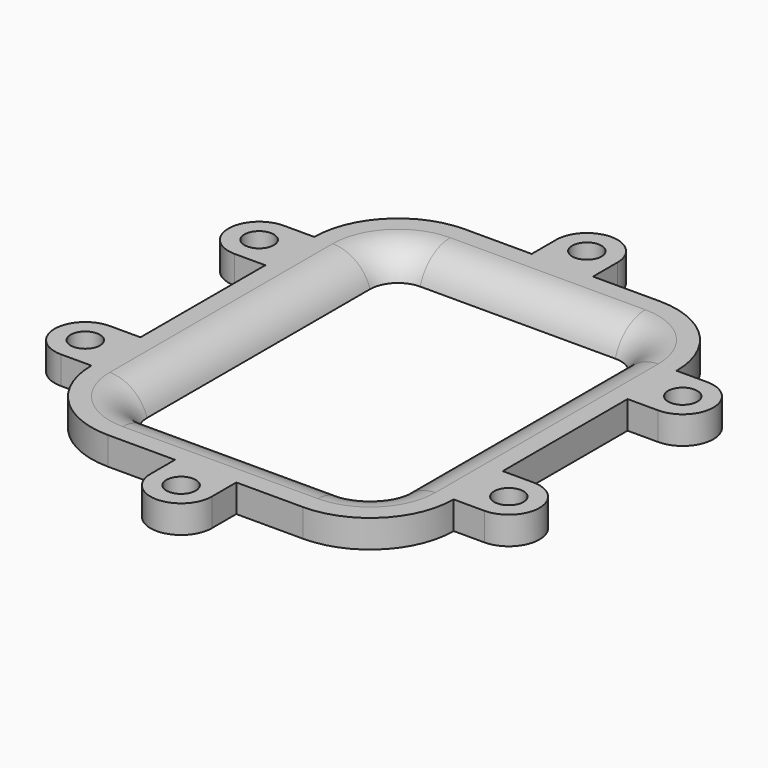
from build123d import *

# Parameters (mm, degrees)
F1_DEPTH     = 5
F3_D         = 5.25
F3_DEPTH     = 40
F3_TIP       = 1.5772591249
F4_T1_DEPTH  = 50
F4_T3_DEPTH  = 35
F4_T6_ANGLE  = 90
F4_T8_ANGLE  = 90
F4_T10_ANGLE = 90
F4_T12_ANGLE = 90


# Not quite as in the source:
# - a fillet or chamfer that OpenCascade refuses, or shapes differently, is made with other operations: its cross-section is extruded or revolved along the edge and cut away or added


with BuildPart() as f1:
    # F0 (on Top) → F1 (new body)
    with BuildSketch(Plane.XY):
        with BuildLine():
            Line((-38, -25), (-32.5, -25))
            ThreePointArc((-32.5, -25), (-28.1066017178, -35.6066017178), (-17.5, -40))
            Line((-17.5, -40), (-5.5, -40))
            Line((-5.5, -40), (-5.5, -45.5))
            ThreePointArc((-5.5, -45.5), (0, -51), (5.5, -45.5))
            Line((5.5, -45.5), (5.5, -40))
            Line((5.5, -40), (17.5, -40))
            ThreePointArc((17.5, -40), (28.1066017178, -35.6066017178), (32.5, -25))
            Line((32.5, -25), (38, -25))
            ThreePointArc((38, -25), (43.5, -19.5), (38, -14))
            Line((38, -14), (32.5, -14))
            Line((32.5, -14), (32.5, 14))
            Line((32.5, 14), (38, 14))
            ThreePointArc((38, 14), (43.5, 19.5), (38, 25))
            Line((38, 25), (32.5, 25))
            ThreePointArc((32.5, 25), (28.1066017178, 35.6066017178), (17.5, 40))
            Line((17.5, 40), (5.5, 40))
            Line((5.5, 40), (5.5, 45.5))
            ThreePointArc((5.5, 45.5), (0, 51), (-5.5, 45.5))
            Line((-5.5, 45.5), (-5.5, 40))
            Line((-5.5, 40), (-17.5, 40))
            ThreePointArc((-17.5, 40), (-28.1066017178, 35.6066017178), (-32.5, 25))
            Line((-32.5, 25), (-38, 25))
            ThreePointArc((-38, 25), (-43.5, 19.5), (-38, 14))
            Line((-38, 14), (-32.5, 14))
            Line((-32.5, 14), (-32.5, -14))
            Line((-32.5, -14), (-38, -14))
            ThreePointArc((-38, -14), (-43.5, -19.5), (-38, -25))
        make_face()
        with BuildLine():
            Line((17.5, -30), (-17.5, -30))
            ThreePointArc((-17.5, -30), (-21.0355339059, -28.5355339059), (-22.5, -25))
            Line((-22.5, -25), (-22.5, 25))
            ThreePointArc((-22.5, 25), (-21.0355339059, 28.5355339059), (-17.5, 30))
            Line((-17.5, 30), (17.5, 30))
            ThreePointArc((17.5, 30), (21.0355339059, 28.5355339059), (22.5, 25))
            Line((22.5, 25), (22.5, -25))
            ThreePointArc((22.5, -25), (21.0355339059, -28.5355339059), (17.5, -30))
        make_face(mode=Mode.SUBTRACT)
    extrude(amount=F1_DEPTH)

    # F3
    with Locations(Plane.XY.offset(5)):
        with Locations((-38, 19.5), (0, 45.5), (38, 19.5), (38, -19.5), (0, -45.5), (-38, -19.5)):
            Hole(F3_D / 2, depth=F3_DEPTH)
            with Locations((0, 0, -(F3_DEPTH + F3_TIP / 2))):  # 118° drill point
                Cone(0, F3_D / 2, F3_TIP, mode=Mode.SUBTRACT)

    # F4: fillet of radius 7 on 1 edges, made by hand

    # F4_s2 → F4_t1 (cut)
    with BuildSketch(Plane.XZ.offset(-25)):
        with BuildLine():
            ThreePointArc((-29.2082039325, 5), (-25.0249037998, 3.6124860802), (-22.5, 0))
            Line((-22.5, 0), (-22.5, 5))
            Line((-22.5, 5), (-29.2082039325, 5))
        make_face()
        with BuildLine():
            ThreePointArc((29.2082039325, 5), (25.0249037998, 3.6124860802), (22.5, 0))
            Line((22.5, 0), (22.5, 5))
            Line((22.5, 5), (29.2082039325, 5))
        make_face()
    extrude(amount=F4_T1_DEPTH, mode=Mode.SUBTRACT)

    # F4_s4 → F4_t3 (cut)
    with BuildSketch(Plane.YZ.offset(-17.5)):
        with BuildLine():
            ThreePointArc((36.7082039325, 5), (32.5249037998, 3.6124860802), (30, 0))
            Line((30, 0), (30, 5))
            Line((30, 5), (36.7082039325, 5))
        make_face()
        with BuildLine():
            ThreePointArc((-36.7082039325, 5), (-32.5249037998, 3.6124860802), (-30, 0))
            Line((-30, 0), (-30, 5))
            Line((-30, 5), (-36.7082039325, 5))
        make_face()
    extrude(amount=F4_T3_DEPTH, mode=Mode.SUBTRACT)

    # F4_s5 → F4_t6 (revolve, cut)
    with BuildSketch(Plane.YZ.offset(-17.5)):
        with BuildLine():
            ThreePointArc((-36.7082039325, 5), (-32.5249037998, 3.6124860802), (-30, 0))
            Line((-30, 0), (-30, 5))
            Line((-30, 5), (-36.7082039325, 5))
        make_face()
    revolve(axis=Axis((-17.5, -25, 5), (0, 0, -1)), revolution_arc=F4_T6_ANGLE, mode=Mode.SUBTRACT)

    # F4_s7 → F4_t8 (revolve, cut)
    with BuildSketch(Plane.XZ.offset(-25)):
        with BuildLine():
            ThreePointArc((-29.2082039325, 5), (-25.0249037998, 3.6124860802), (-22.5, 0))
            Line((-22.5, 0), (-22.5, 5))
            Line((-22.5, 5), (-29.2082039325, 5))
        make_face()
    revolve(axis=Axis((-17.5, 25, 5), (0, 0, -1)), revolution_arc=F4_T8_ANGLE, mode=Mode.SUBTRACT)

    # F4_s9 → F4_t10 (revolve, cut)
    with BuildSketch(Plane.YZ.offset(17.5)):
        with BuildLine():
            ThreePointArc((36.7082039325, 5), (32.5249037998, 3.6124860802), (30, 0))
            Line((30, 0), (30, 5))
            Line((30, 5), (36.7082039325, 5))
        make_face()
    revolve(axis=Axis((17.5, 25, 5), (0, 0, -1)), revolution_arc=F4_T10_ANGLE, mode=Mode.SUBTRACT)

    # F4_s11 → F4_t12 (revolve, cut)
    with BuildSketch(Plane.XZ.offset(25)):
        with BuildLine():
            ThreePointArc((29.2082039325, 5), (25.0249037998, 3.6124860802), (22.5, 0))
            Line((22.5, 0), (22.5, 5))
            Line((22.5, 5), (29.2082039325, 5))
        make_face()
    revolve(axis=Axis((17.5, -25, 5), (0, 0, -1)), revolution_arc=F4_T12_ANGLE, mode=Mode.SUBTRACT)


solid = f1.part
